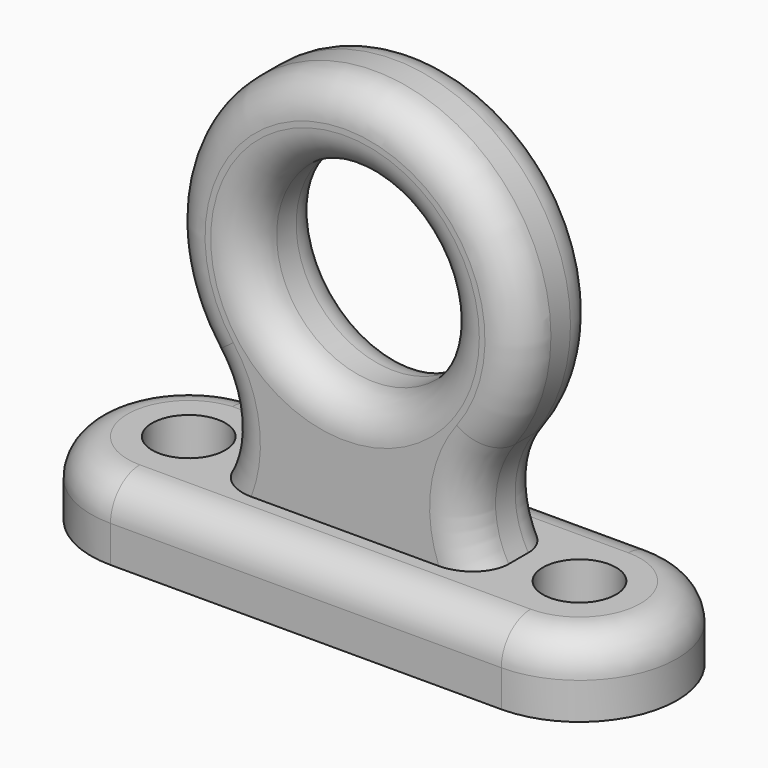
from build123d import *

# Parameters (mm, degrees)
F0_R     = 1.5
F1_DEPTH = 3
F2_R     = 4
F3_DEPTH = 2
F4_R     = 1.5


# Not quite as in the source:
# - a feature names something its author has since deleted; it is built from what else it names


with BuildPart() as f1:
    # F0 (on Top) → F1 (new body)
    with BuildSketch(Plane.XY):
        with BuildLine():
            Line((7.9999998792, 3.9986097976), (-8.2109180559, 3.9986097976))
            ThreePointArc((-8.2109180559, 3.9986097976), (-12.0013898401, -0.104105532), (-7.9999998792, -4.0013902024))
            Line((-7.9999998792, -4.0013902024), (7.9999998792, -4.0013902024))
            ThreePointArc((7.9999998792, -4.0013902024), (11.9999998792, -0.0013902024), (7.9999998792, 3.9986097976))
        make_face()
        with Locations((-7.9999998792, 0.0013902024)):
            Circle(F0_R, mode=Mode.SUBTRACT)
        with Locations((7.9999998792, -0.0013902024)):
            Circle(F0_R, mode=Mode.SUBTRACT)
    extrude(amount=F1_DEPTH)

    # F2 (on Front) → F3 (join, symmetric)
    with BuildSketch(Plane.XZ):
        with BuildLine():
            Line((-5.5, 3), (5.5, 3))
            ThreePointArc((5.5, 3), (4.9716755174, 5.2460362856), (5.7717823496, 7.4102069842))
            ThreePointArc((5.7717823496, 7.4102069842), (0, 19), (-5.7717823496, 7.4102069842))
            ThreePointArc((-5.7717823496, 7.4102069842), (-4.9716755174, 5.2460362856), (-5.5, 3))
        make_face()
        with Locations((0, 11.7679133954)):
            Circle(F2_R, mode=Mode.SUBTRACT)
    extrude(amount=F3_DEPTH, both=True)

    # F4
    f4_edges = [f1.edges().sort_by_distance(p)[0] for p in [
        (0, -2, 19),
        (0, 2, 19),
        (0, -4.00139, 3),
        (-4, -2, 11.767913),
        (-4, 2, 11.767913),
    ]]
    fillet(f4_edges, radius=F4_R)


solid = f1.part
